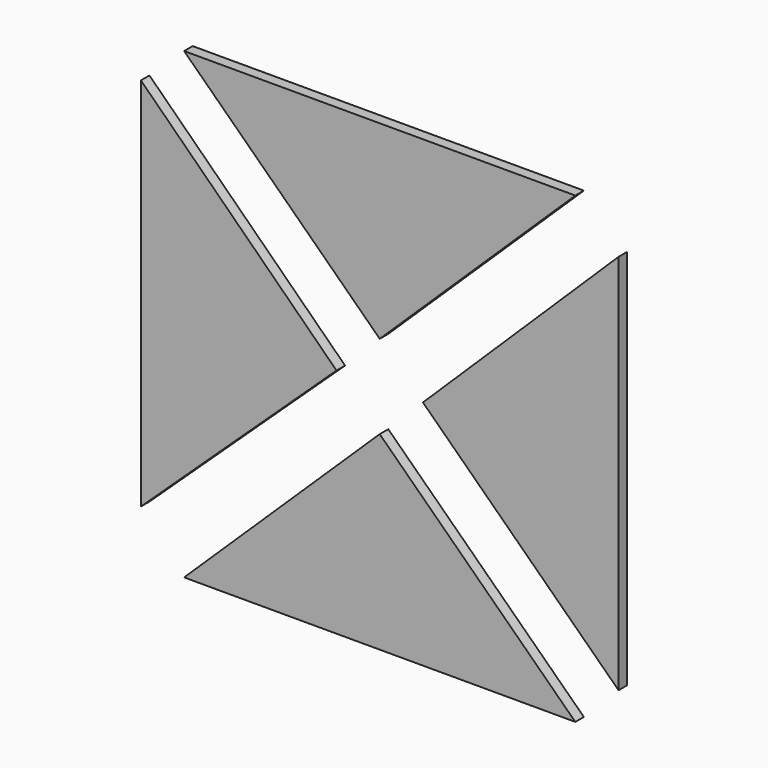
from build123d import *

# Parameters (mm, degrees)
F1_DEPTH = 1.5


# Not quite as in the source:
# - a feature names something its author has since deleted; it is built from what else it names


with BuildPart() as f1:
    # F0 (on Front) → F1 (new body)
    with BuildSketch(Plane.XZ):
        Polygon((-10.6868883812, -13.0220385311), (-65.5616819859, -13.0220385311), (-38.1242851835, -39.6404085632), align=None)
    extrude(amount=F1_DEPTH)


with BuildPart() as f1b:
    # F0 (on Front) → F1, piece 2 (new body)
    with BuildSketch(Plane.XZ):
        Polygon((-38.1242851835, -51.403668499), (-65.5616819859, -78.0220385311), (-10.6868883812, -78.0220385311), align=None)
    extrude(amount=F1_DEPTH)


with BuildPart() as f1c:
    # F0 (on Front) → F1, piece 3 (new body)
    with BuildSketch(Plane.XZ):
        Polygon((-4.6242851835, -72.1404085632), (-4.6242851835, -18.6169743538), (-32.0616819859, -45.5220385311), align=None)
    extrude(amount=F1_DEPTH)


with BuildPart() as f1d:
    # F0 (on Front) → F1, piece 4 (new body)
    with BuildSketch(Plane.XZ):
        Polygon((-44.1868883812, -45.5220385311), (-71.6242851835, -18.6169743538), (-71.6242851835, -71.2447017431), align=None)
    extrude(amount=F1_DEPTH)


solid = Compound([f1.part, f1b.part, f1c.part, f1d.part])
